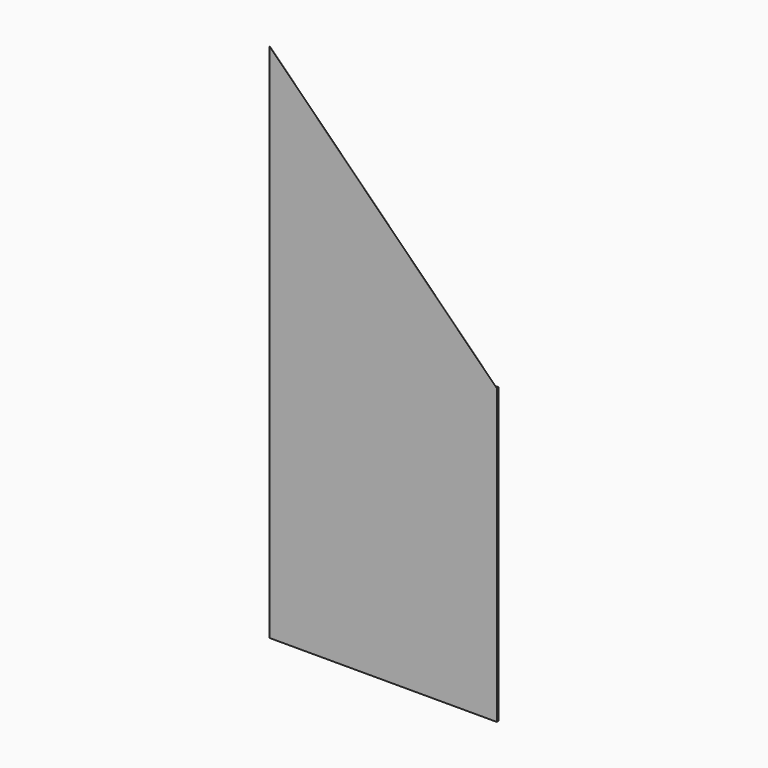
from build123d import *

# Parameters (mm, degrees)
F1_DEPTH = 4
F2_SIZE  = 3.99999
F4_DEPTH = 25


# Not quite as in the source:
# - a fillet or chamfer is up to 0.001 mm smaller than in the source, because OpenCascade refuses the exact size
# - ends of sketch curves that miss each other by under 0.0002 mm in the source are joined


with BuildPart() as f1:
    # F0 (on Front) → F1 (new body)
    with BuildSketch(Plane.XZ):
        Polygon((0, 944.56), (0, 0), (412.03, 0), (412.03, 532.53), align=None)
    extrude(amount=F1_DEPTH)

    # F2 (size 4 in the source; OpenCascade refuses exactly that, so slightly less here)
    f2_edges = [f1.edges().sort_by_distance(p)[0] for p in [
        (206.015, 0, 738.545),
    ]]
    chamfer(f2_edges, length=F2_SIZE)

    # F3 (on face) → F4 (join)
    with BuildSketch(Plane.YZ.offset(412.03)):
        Polygon((-3.99999, 532.53), (0, 526.8731598926), (0, 532.53), align=None)
    extrude(amount=-F4_DEPTH)


solid = f1.part
